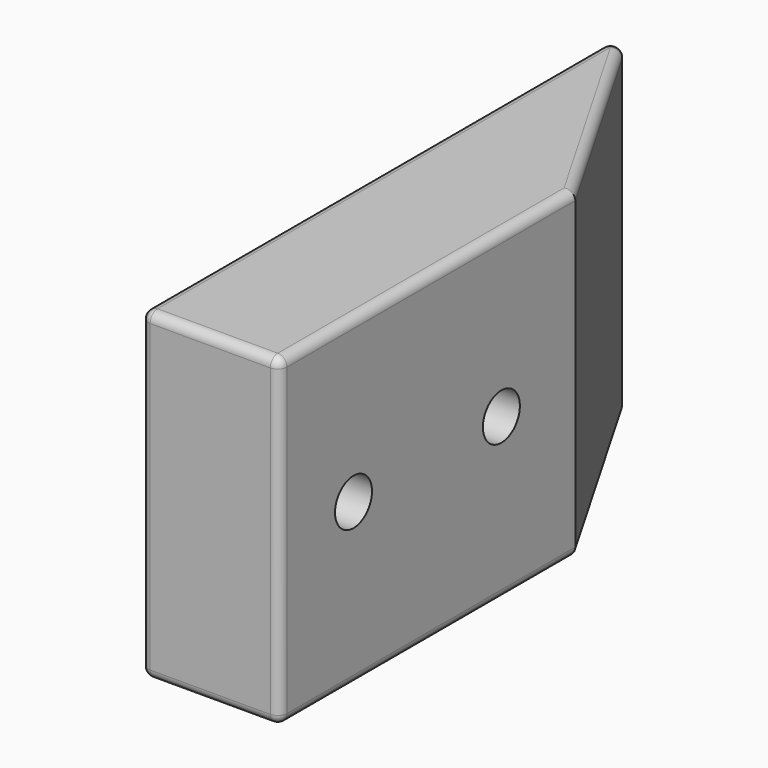
from build123d import *

# Parameters (mm, degrees)
F1_DEPTH       = 44.45
F3_D           = 6.35
F3_CSINK_D     = 10.16
F3_CSINK_ANGLE = 82
F4_T1_DEPTH    = 68.1485226281
F5_R           = 1.27


# Not quite as in the source:
# - a fillet or chamfer that OpenCascade refuses, or shapes differently, is made with other operations: its cross-section is extruded or revolved along the edge and cut away or added
# - a feature names something its author has since deleted; it is built from what else it names


with BuildPart() as f1:
    # F0 (on Top) → F1 (new body)
    with BuildSketch(Plane.XY):
        Polygon((0, 83.7955678842), (0, 0), (19.05, 0), (19.05, 50.8), align=None)
    extrude(amount=F1_DEPTH)

    # F3 (through all)
    with Locations(Plane(origin=(0, 0, 0), x_dir=(0, -1, 0), z_dir=(-1, 0, 0))):
        with Locations((-12.7, 22.225), (-38.1, 22.225)):
            CounterSinkHole(F3_D / 2, F3_CSINK_D / 2, counter_sink_angle=F3_CSINK_ANGLE)

    # F4: fillet of radius 1.27 on 1 edges, made by hand

    # F4_s2 → F4_t1 (cut)
    with BuildSketch(Plane.XY.offset(-11.849261314)):
        with BuildLine():
            ThreePointArc((0, 79.0558633586), (0.9412998127, 80.282589158), (2.3698522628, 79.6908633586))
            Line((2.3698522628, 79.6908633586), (0, 83.7955678842))
            Line((0, 83.7955678842), (0, 79.0558633586))
        make_face()
    extrude(amount=F4_T1_DEPTH, mode=Mode.SUBTRACT)

    # F5
    f5_edges = [f1.edges().sort_by_distance(p)[0] for p in [
        (0.9413, 80.282589, 44.45),
        (10.709926, 65.245432, 44.45),
        (19.05, 25.4, 44.45),
        (9.525, 0, 44.45),
        (0, 39.527932, 44.45),
        (0.9413, 80.282589, 0),
        (10.709926, 65.245432, 0),
        (19.05, 25.4, 0),
        (9.525, 0, 0),
        (0, 39.527932, 0),
        (0, 0, 22.225),
        (19.05, 0, 22.225),
    ]]
    fillet(f5_edges, radius=F5_R)


solid = f1.part
